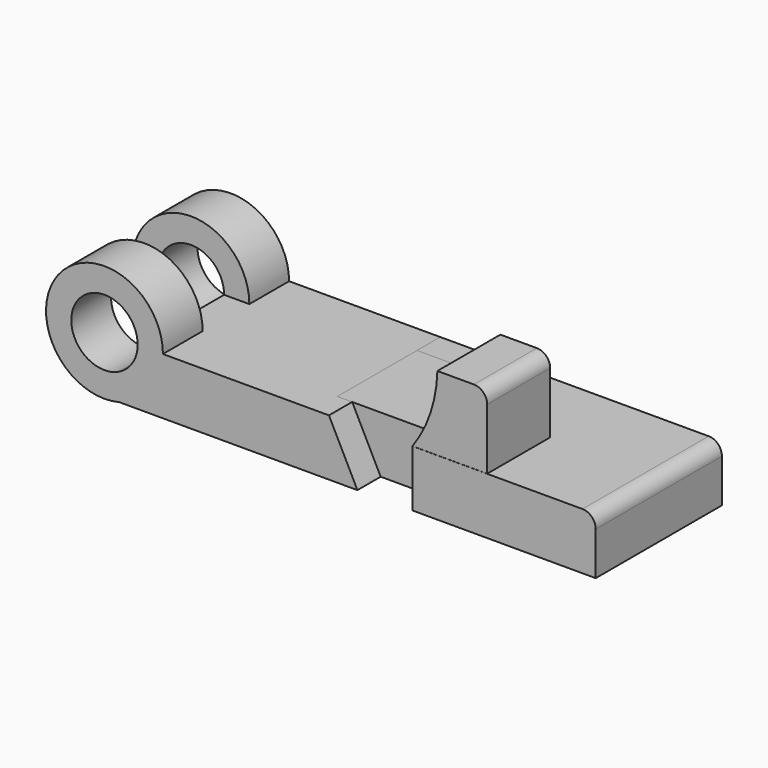
from build123d import *

# Parameters (mm, degrees)
F1_DEPTH = 30.1625
F3_DEPTH = 19.05
F4_R     = 5.08
F5_DEPTH = 30.1092732698
F6_R     = 5.08
F7_DEPTH = 11.1207123846
F8_DEPTH = 11.1633


# Not quite as in the source:
# - a feature names something its author has since deleted; it is built from what else it names


with BuildPart() as f1:
    # F0 (on Front) → F1 (new body, symmetric)
    with BuildSketch(Plane.XZ):
        with BuildLine():
            Line((98.0956078965, 0), (34.5956078965, 0))
            ThreePointArc((34.5956078965, 0), (29.9165165739, -13.6850357282), (17.838252592, -21.6405141975))
            Line((17.838252592, -21.6405141975), (108.9896394755, -21.6405141975))
            Line((108.9896394755, -21.6405141975), (98.0956078965, 0))
        make_face()
        with BuildLine():
            Line((34.5956078965, 0), (24.9436078965, 0))
            ThreePointArc((24.9436078965, 0), (23.0218727762, -6.7170682729), (17.838252592, -11.4013135529))
            Line((17.838252592, -11.4013135529), (17.838252592, -21.6405141975))
            ThreePointArc((17.838252592, -21.6405141975), (29.9165165739, -13.6850357282), (34.5956078965, 0))
        make_face()
        with BuildLine():
            ThreePointArc((17.838252592, -11.4013135529), (1.4653430168, 6.7170682729), (24.9436078965, 0))
            Line((24.9436078965, 0), (34.5956078965, 0))
            ThreePointArc((34.5956078965, 0), (-5.4293007808, 13.6850357282), (17.838252592, -21.6405141975))
            Line((17.838252592, -21.6405141975), (17.838252592, -11.4013135529))
        make_face()
    extrude(amount=F1_DEPTH, both=True)

    # F0 (on Front) → F8 (cut, symmetric)
    with BuildSketch(Plane.XZ):
        with BuildLine():
            ThreePointArc((17.838252592, -11.4013135529), (1.4653430168, 6.7170682729), (24.9436078965, 0))
            Line((24.9436078965, 0), (34.5956078965, 0))
            ThreePointArc((34.5956078965, 0), (-5.4293007808, 13.6850357282), (17.838252592, -21.6405141975))
            Line((17.838252592, -21.6405141975), (17.838252592, -11.4013135529))
        make_face()
    extrude(amount=F8_DEPTH, both=True, mode=Mode.SUBTRACT)


with BuildPart() as f1b:
    # F0 (on Front) → F1, piece 2 (new body, symmetric)
    with BuildSketch(Plane.XZ):
        Polygon((130.004652592, 0), (130.004652592, -21.6405141975), (200.1410263589, -21.6405141975), (200.1410263589, 0), (158.579652592, 0), align=None)
    extrude(amount=F1_DEPTH, both=True)

    # F4
    f4_edges = [f1b.edges().sort_by_distance(p)[0] for p in [
        (200.141026, 0, 0),
    ]]
    fillet(f4_edges, radius=F4_R)


with BuildPart() as f3:
    # F2 (on Front) → F3 (new body, symmetric)
    with BuildSketch(Plane.XZ):
        Polygon((131.5081966538, 0), (92.4129226052, 0), (92.4129226052, -21.6405141975), (131.5088617504, -21.6405141975), (131.5088617504, 0), align=None)
    extrude(amount=F3_DEPTH, both=True)


with BuildPart() as f5:
    # F0 (on Front) → F5 (new body)
    with BuildSketch(Plane.XZ):
        with BuildLine():
            ThreePointArc((139.529652592, 28.3959060907), (136.9074278137, 13.4800283762), (130.004652592, 0))
            Line((130.004652592, 0), (158.579652592, 0))
            Line((158.579652592, 0), (158.579652592, 28.3959060907))
            Line((158.579652592, 28.3959060907), (139.529652592, 28.3959060907))
        make_face()
    extrude(amount=F5_DEPTH)

    # F6
    f6_edges = [f5.edges().sort_by_distance(p)[0] for p in [
        (158.579653, -15.054637, 28.395906),
    ]]
    fillet(f6_edges, radius=F6_R)


with BuildPart() as f7:
    # F7 (new): a face of the model
    f7_faces = [f3.part.faces().sort_by_distance(p)[0] for p in [
        (111.9608921778, 19.05, -10.8202570987),
    ]]
    extrude(f7_faces, amount=F7_DEPTH)


solid = Compound([f1.part, f1b.part, f3.part, f5.part, f7.part])
